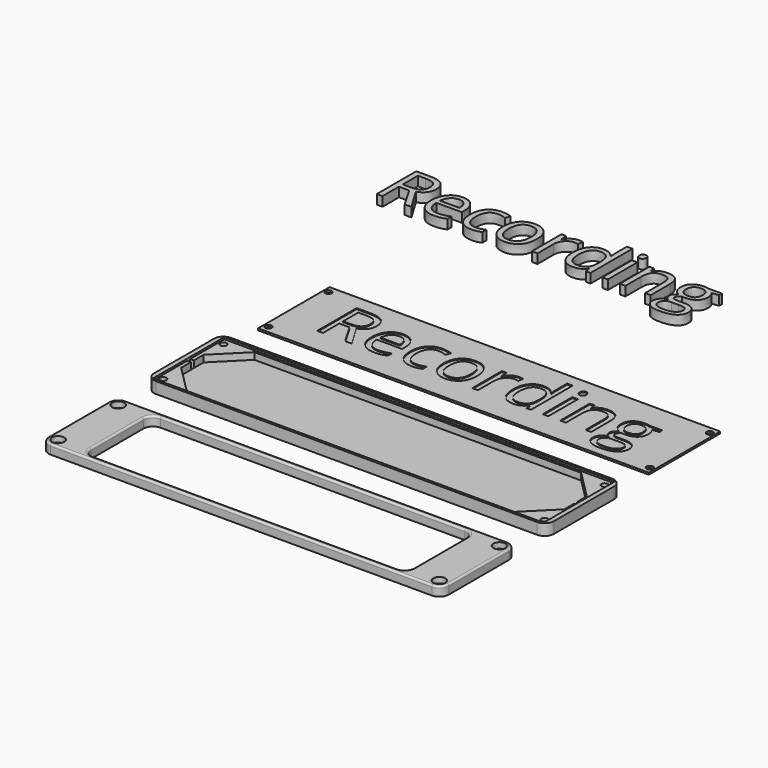
from build123d import *

# Parameters (mm, degrees)
F0_W            = 213
F0_H            = 50
F1_DEPTH        = 5
F2_DEPTH        = 1.4
F3_W            = 213
F3_H            = 50
F4_DEPTH        = 1
F6_D            = 3.4
F6_DEPTH        = 7
F6_TIP          = 1.0214630523
F7_R            = 5
F8_W            = 213
F8_H            = 50
F8_W_2          = 172
F8_H_2          = 45
F9_DEPTH        = 5
F11_D           = 3.4
F11_DEPTH       = 5
F11_CBORE_D     = 6.5
F11_CBORE_DEPTH = 3
F11_TIP         = 1.0214630523
F12_R           = 5
F13_R           = 1
F14_W           = 208
F14_H           = 47.5
F15_DEPTH       = 1
F17_D           = 3.4
F17_DEPTH       = 1
F17_TIP         = 1.0214630523
F18_TEXT_SIZE   = 36.7403497196
F19_DEPTH       = 0.5
F20_TEXT_SIZE   = 36.7403497196
F21_DEPTH       = 5


# Not quite as in the source:
# - Text() gives the source's letters only with a copy of the font that has no kerning and outlines rounded to 1/6400 em; it was checked with that copy


with BuildPart() as f1:
    # F0 (on Top) → F1 (new body)
    with BuildSketch(Plane.XY):
        with Locations((0, -22.5)):
            Rectangle(F0_W, F0_H)
        Polygon((-87, 0), (0, 0), (87, 0), (102, -15), (102, -21.5), (104, -21.5), (104, -23.5), (102, -23.5), (102, -30), (87, -45), (0, -45), (-87, -45), (-102, -30), (-102, -23.5), (-104, -23.5), (-104, -21.5), (-102, -21.5), (-102, -15), align=None, mode=Mode.SUBTRACT)
    extrude(amount=F1_DEPTH)

    # F0 (on Top) → F2 (join)
    with BuildSketch(Plane.XY):
        Polygon((87, 0), (0, 0), (-87, 0), (-102, -15), (-102, -21.5), (-102, -23.5), (-102, -30), (-87, -45), (0, -45), (87, -45), (102, -30), (102, -23.5), (102, -21.5), (102, -15), align=None)
    extrude(amount=F2_DEPTH)

    # F3 (on face) → F4 (join)
    with BuildSketch(Plane.XY.offset(5)):
        with Locations((0, -22.5)):
            Rectangle(F3_W, F3_H)
        Polygon((-104, -21.5), (-104, 1.25), (104, 1.25), (104, -21.5), (104, -23.5), (104, -46.25), (-104, -46.25), (-104, -23.5), align=None, mode=Mode.SUBTRACT)
    extrude(amount=F4_DEPTH)

    # F6
    with Locations(Plane.XY.offset(6)):
        with Locations((-101.5, -2.5), (-101.5, -42.5), (101.5, -42.5), (101.5, -2.5)):
            Hole(F6_D / 2, depth=F6_DEPTH)
            with Locations((0, 0, -(F6_DEPTH + F6_TIP / 2))):  # 118° drill point
                Cone(0, F6_D / 2, F6_TIP, mode=Mode.SUBTRACT)

    # F7
    f7_edges = [f1.edges().sort_by_distance(p)[0] for p in [
        (-106.5, 2.5, 3),
        (-106.5, -47.5, 3),
        (106.5, -47.5, 3),
        (106.5, 2.5, 3),
    ]]
    fillet(f7_edges, radius=F7_R)


with BuildPart() as f9:
    # F8 (on Top) → F9 (new body)
    with BuildSketch(Plane.XY):
        with Locations((0, -92.5)):
            Rectangle(F8_W, F8_H)
        with Locations((0, -92.5)):
            Rectangle(F8_W_2, F8_H_2, mode=Mode.SUBTRACT)
    extrude(amount=F9_DEPTH)

    # F11
    with Locations(Plane.XY.offset(5)):
        with Locations((-101.5, -72.5), (-101.5, -112.5), (101.5, -72.5), (101.5, -112.5)):
            CounterBoreHole(F11_D / 2, F11_CBORE_D / 2, F11_CBORE_DEPTH, depth=F11_DEPTH)
            with Locations((0, 0, -(F11_DEPTH + F11_TIP / 2))):  # 118° drill point
                Cone(0, F11_D / 2, F11_TIP, mode=Mode.SUBTRACT)

    # F12
    f12_edges = [f9.edges().sort_by_distance(p)[0] for p in [
        (-86, -70, 2.5),
        (-86, -115, 2.5),
        (86, -70, 2.5),
        (86, -115, 2.5),
        (106.5, -117.5, 2.5),
        (106.5, -67.5, 2.5),
        (-106.5, -117.5, 2.5),
        (-106.5, -67.5, 2.5),
    ]]
    fillet(f12_edges, radius=F12_R)

    # F13
    f13_edges = [f9.edges().sort_by_distance(p)[0] for p in [
        (0, -70, 5),
        (0, -67.5, 5),
    ]]
    fillet(f13_edges, radius=F13_R)


with BuildPart() as f15:
    # F14 (on Top) → F15 (new body)
    with BuildSketch(Plane.XY):
        with Locations((0, 47.5)):
            Rectangle(F14_W, F14_H)
    extrude(amount=F15_DEPTH)

    # F17
    with Locations(Plane.XY.offset(1)):
        with Locations((-101.5, 67.5), (-101.5, 27.5), (101.5, 27.5), (101.5, 67.5)):
            Hole(F17_D / 2, depth=F17_DEPTH)
            with Locations((0, 0, -(F17_DEPTH + F17_TIP / 2))):  # 118° drill point
                Cone(0, F17_D / 2, F17_TIP, mode=Mode.SUBTRACT)

    # F18 (on face) → F19 (cut)
    with BuildSketch(Plane.XY.offset(1)):
        with Locations((-87, 37.2969482019)):
            Text('Recording', F18_TEXT_SIZE, font='Open Sans', text_align=(TextAlign.LEFT, TextAlign.BOTTOM))
    extrude(amount=-F19_DEPTH, mode=Mode.SUBTRACT)


with BuildPart() as f21:
    # F20 (on Top) → F21 (new body)
    with BuildSketch(Plane.XY):
        with Locations((-139.8132356703, 142.9795596674)):
            Text('Recording', F20_TEXT_SIZE, font='Open Sans', text_align=(TextAlign.LEFT, TextAlign.BOTTOM))
    extrude(amount=F21_DEPTH)


solid = Compound([f1.part, f9.part, f15.part, f21.part])
